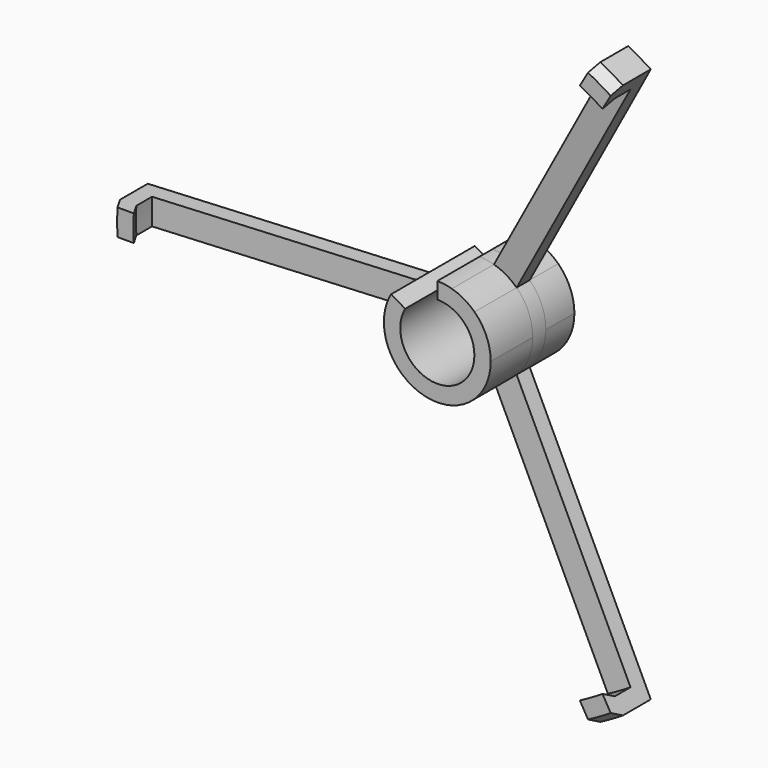
from build123d import *
from build123d import SkipClean  # not in build123d's __all__

# Parameters (mm, degrees)
F3_DEPTH = 25.4


with BuildPart() as f1:
    # F0 (on Top) → F1 (revolve)
    with BuildSketch(Plane.XY):
        Polygon((63.7286, -3.81), (63.7286, 2.9399013527), (10.3759, 7.0484601322), (10.3759, 13.97), (7.2009, 13.97), (7.2009, -6.35), (10.3759, -6.35), (10.3759, 3.8640599232), (60.5536, 0), (60.5536, -3.81), (59.2836, -6.0097045256), (62.4586, -6.0097045256), align=None)
    revolve(axis=Axis((0, -13.2026916835, 0), (0, -1, 0)))

    # F2 (on face) → F3 (cut)
    with BuildSketch(Plane(origin=(0, 13.97, 0), x_dir=(-1, 0, 0), z_dir=(0, 1, 0))):
        with BuildLine():
            Line((111.0251099892, -2.54), (10.0602038155, -2.54))
            ThreePointArc((10.0602038155, -2.54), (5.18795, -8.9857929871), (-2.8303973822, -9.9823920715))
            Line((-2.8303973822, -9.9823920715), (-53.312850469, -97.4205657086))
            ThreePointArc((-53.312850469, -97.4205657086), (40.7588842751, -70.5964584242), (111.0251099892, -2.54))
        make_face()
        with BuildLine():
            Line((10.0602038155, 2.54), (111.0251099892, 2.54))
            ThreePointArc((111.0251099892, 2.54), (40.7588842751, 70.5964584242), (-53.312850469, 97.4205657086))
            Line((-53.312850469, 97.4205657086), (-2.8303973822, 9.9823920715))
            ThreePointArc((-2.8303973822, 9.9823920715), (-1.4288105045, 10.2770521723), (0, 10.3759))
            Line((0, 10.3759), (0, 0))
            Line((0, 0), (8.9857929871, 5.18795))
            ThreePointArc((8.9857929871, 5.18795), (9.6145935095, 3.9011398921), (10.0602038155, 2.54))
        make_face()
        with BuildLine():
            Line((-7.2298064334, 7.4423920715), (-57.7122595202, 94.8805657086))
            ThreePointArc((-57.7122595202, 94.8805657086), (-81.5177685501, 0), (-57.7122595202, -94.8805657086))
            Line((-57.7122595202, -94.8805657086), (-7.2298064334, -7.4423920715))
            ThreePointArc((-7.2298064334, -7.4423920715), (-10.3759, 0), (-7.2298064334, 7.4423920715))
        make_face()
    with SkipClean():  # cleaning this boolean's faces spoils the solid; the shape is the same uncleaned
        extrude(amount=-F3_DEPTH, mode=Mode.SUBTRACT)


solid = f1.part
